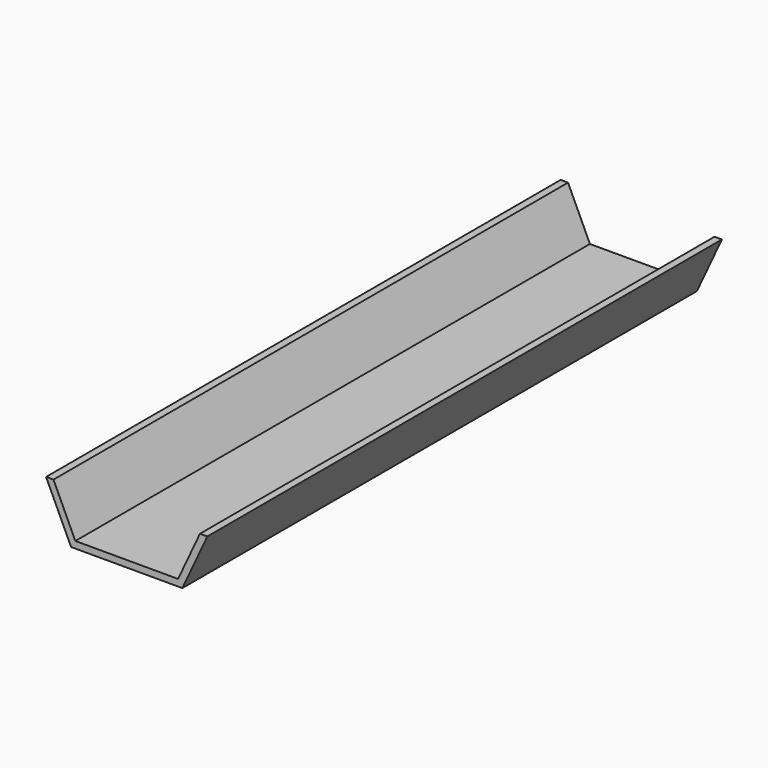
from build123d import *

# Parameters (mm, degrees)
F1_DEPTH = 304.8


# Not quite as in the source:
# - ends of sketch curves that miss each other by under 0.0002 mm in the source are joined


with BuildPart() as f1:
    # F0 (on Front) → F1 (new body)
    with BuildSketch(Plane.XZ):
        Polygon((-39.22352381, 12.7743089993), (-27.3793092929, -12.6256910007), (25.3481481273, -12.6256910007), (37.1923626445, 12.7743089993), (33.6891880845, 12.7744169383), (23.3254500493, -9.4506910007), (-25.3566112148, -9.4506910007), (-35.7203079071, 12.7743282779), align=None)
    extrude(amount=F1_DEPTH)


solid = f1.part
